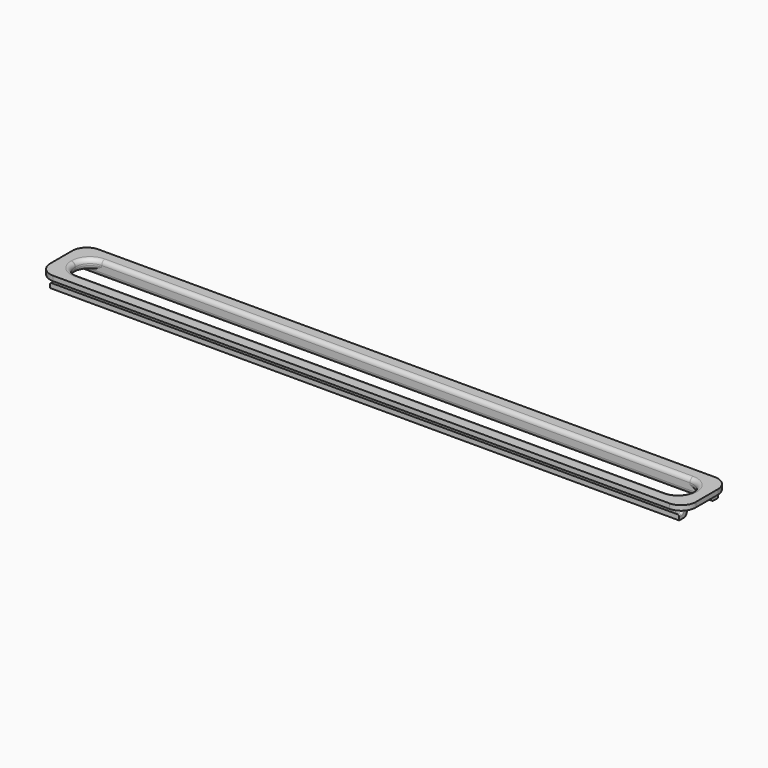
from build123d import *

# Parameters (mm, degrees)
F0_W         = 155
F0_H         = 10
F0_W_2       = 152.0637926605
F0_H_2       = 7.2836262298
F1_DEPTH     = 1.2
F2_W         = 159
F2_H         = 14
F2_W_2       = 155
F2_H_2       = 10
F2_W_3       = 152.0637926605
F2_H_3       = 7.2836262298
F3_DEPTH     = 1.2
F4_W         = 155
F4_H         = 1
F5_DEPTH     = 1.2
F6_R         = 3.6
F7_T1_DEPTH  = 160
F7_T3_DEPTH  = 0.0836262298
F7_T5_DEPTH  = 144.8637926605
F7_T10_ANGLE = 129.8047192326
F7_T13_ANGLE = 90
F7_T17_ANGLE = 129.8047192326
F7_T22_ANGLE = 129.8047192326
F7_T25_ANGLE = 90
F7_T27_ANGLE = 90
F7_T29_ANGLE = 90
F7_T33_ANGLE = 129.8047192326
F8_F1_R      = 0.5
F8_F2_R      = 0.5
F8_F3_R      = 0.5


# Not quite as in the source:
# - a fillet or chamfer that OpenCascade refuses, or shapes differently, is made with other operations: its cross-section is extruded or revolved along the edge and cut away or added


with BuildPart() as f1:
    # F0 (on Top) → F1 (new body)
    with BuildSketch(Plane.XY):
        with Locations((77.5, 5)):
            Rectangle(F0_W, F0_H)
        with Locations((77.5, 5)):
            Rectangle(F0_W_2, F0_H_2, mode=Mode.SUBTRACT)
    extrude(amount=F1_DEPTH)

    # F2 (on face) → F3 (join)
    with BuildSketch(Plane.XY.offset(1.2)):
        with Locations((77.5, 5)):
            Rectangle(F2_W, F2_H)
        with Locations((77.5, 5)):
            Rectangle(F2_W_2, F2_H_2, mode=Mode.SUBTRACT)
        with Locations((77.5, 5)):
            Rectangle(F2_W_2, F2_H_2)
        with Locations((77.5, 5)):
            Rectangle(F2_W_3, F2_H_3, mode=Mode.SUBTRACT)
    extrude(amount=F3_DEPTH)

    # F4 (on face) → F5 (join)
    with BuildSketch(Plane(origin=(0, 0, 0), x_dir=(1, 0, 0), z_dir=(0, 0, -1))):
        with Locations((77.5, 0.5)):
            Rectangle(F4_W, F4_H)
        Polygon((155, -1.3581868851), (155, 0), (0, 0), (0, -1.3581868851), (1.4681036697, -1.3581868851), (153.5318963303, -1.3581868851), align=None)
        Polygon((155, -10), (155, -8.6418131149), (153.5318963303, -8.6418131149), (1.4681036697, -8.6418131149), (0, -8.6418131149), (0, -10), align=None)
        with Locations((77.5, -10.5)):
            Rectangle(F4_W, F4_H)
    extrude(amount=F5_DEPTH)

    # F6
    f6_edges = [f1.edges().sort_by_distance(p)[0] for p in [
        (1.468104, 1.358187, 1.2),
        (1.468104, 8.641813, 1.2),
        (153.531896, 1.358187, 1.2),
        (153.531896, 8.641813, 1.2),
        (157, -2, 1.8),
        (157, 12, 1.8),
        (-2, 12, 1.8),
        (-2, -2, 1.8),
    ]]
    fillet(f6_edges, radius=F6_R)

    # F7: fillet of radius 1 on 16 edges, made by hand

    # F7_s2 → F7_t1 (cut)
    with BuildSketch(Plane.YZ.offset(-2.5)):
        with BuildLine():
            ThreePointArc((1.3581868851, -0.2), (1.0652936663, -0.9071067812), (0.3581868851, -1.2))
            Line((0.3581868851, -1.2), (1.3581868851, -1.2))
            Line((1.3581868851, -1.2), (1.3581868851, -0.2))
        make_face()
        with BuildLine():
            ThreePointArc((8.6418131149, -0.2), (8.9347063337, -0.9071067812), (9.6418131149, -1.2))
            Line((9.6418131149, -1.2), (8.6418131149, -1.2))
            Line((8.6418131149, -1.2), (8.6418131149, -0.2))
        make_face()
    extrude(amount=F7_T1_DEPTH, mode=Mode.SUBTRACT)

    # F7_s4 → F7_t3 (cut)
    with BuildSketch(Plane.XZ.offset(-5.0418131149)):
        with BuildLine():
            ThreePointArc((0.4681036697, 0), (1.1752104509, 0.2928932188), (1.4681036697, 1))
            Line((1.4681036697, 1), (1.4681036697, 0))
            Line((1.4681036697, 0), (0.4681036697, 0))
        make_face()
        with BuildLine():
            ThreePointArc((1.4681036697, 1.4), (1.1752104509, 2.1071067812), (0.4681036697, 2.4))
            Line((0.4681036697, 2.4), (1.4681036697, 2.4))
            Line((1.4681036697, 2.4), (1.4681036697, 1.4))
        make_face()
        with BuildLine():
            ThreePointArc((154.5318963303, 2.4), (153.8247895491, 2.1071067812), (153.5318963303, 1.4))
            Line((153.5318963303, 1.4), (153.5318963303, 2.4))
            Line((153.5318963303, 2.4), (154.5318963303, 2.4))
        make_face()
        with BuildLine():
            ThreePointArc((154.5318963303, 0), (153.8247895491, 0.2928932188), (153.5318963303, 1))
            Line((153.5318963303, 1), (153.5318963303, 0))
            Line((153.5318963303, 0), (154.5318963303, 0))
        make_face()
    extrude(amount=F7_T3_DEPTH, mode=Mode.SUBTRACT)

    # F7_s6 → F7_t5 (cut)
    with BuildSketch(Plane.YZ.offset(5.0681036697)):
        with BuildLine():
            ThreePointArc((1.3581868851, 1.4), (1.0652936663, 2.1071067812), (0.3581868851, 2.4))
            Line((0.3581868851, 2.4), (1.3581868851, 2.4))
            Line((1.3581868851, 2.4), (1.3581868851, 1.4))
        make_face()
        with BuildLine():
            ThreePointArc((8.6418131149, 1.4), (8.9347063337, 2.1071067812), (9.6418131149, 2.4))
            Line((9.6418131149, 2.4), (8.6418131149, 2.4))
            Line((8.6418131149, 2.4), (8.6418131149, 1.4))
        make_face()
    extrude(amount=F7_T5_DEPTH, mode=Mode.SUBTRACT)


with BuildPart() as f7_tool8:
    # F7_s9 → F7_t10 (revolve)
    with BuildSketch(Plane(origin=(0.5115194158, -0.4262532935, 0), x_dir=(0, 0, 1), z_dir=(0.7682307976, -0.6401729779, 0))):
        with BuildLine():
            ThreePointArc((0, -11.7177391291), (0.2928932188, -11.0106323479), (1, -10.7177391291))
            Line((1, -10.7177391291), (0, -10.7177391291))
            Line((0, -10.7177391291), (0, -11.7177391291))
        make_face()
    revolve(axis=Axis((5.0681036697, 5.0418131149, 0), (0, 0, 1)), revolution_arc=F7_T10_ANGLE)

    split(bisect_by=Plane.XZ.offset(-8.6418131149), keep=Keep.TOP)


with BuildPart() as f1_1:
    add(f1.part)

    # F7_t7: cut F7_tool8
    add(f7_tool8.part, mode=Mode.SUBTRACT)

    # F7_s12 → F7_t13 (revolve, cut)
    with BuildSketch(Plane.YZ.offset(5.0681036697)):
        with BuildLine():
            ThreePointArc((8.6418131149, 1.4), (8.9347063337, 2.1071067812), (9.6418131149, 2.4))
            Line((9.6418131149, 2.4), (8.6418131149, 2.4))
            Line((8.6418131149, 2.4), (8.6418131149, 1.4))
        make_face()
    revolve(axis=Axis((5.0681036697, 5.0418131149, 2.4), (0, 0, 1)), revolution_arc=F7_T13_ANGLE, mode=Mode.SUBTRACT)


with BuildPart() as f7_tool15:
    # F7_s16 → F7_t17 (revolve)
    with BuildSketch(Plane(origin=(90.9661571375, 75.8028393036, 0), x_dir=(0, 0, 1), z_dir=(-0.7682307976, -0.6401729779, 0))):
        with BuildLine():
            ThreePointArc((0, -87.5090724404), (0.2928932188, -88.2161792216), (1, -88.5090724404))
            Line((1, -88.5090724404), (0, -88.5090724404))
            Line((0, -88.5090724404), (0, -87.5090724404))
        make_face()
    revolve(axis=Axis((149.9318963303, 5.0418131149, 0), (0, 0, -1)), revolution_arc=F7_T17_ANGLE)

    split(bisect_by=Plane.XZ.offset(-8.6418131149), keep=Keep.TOP)


with BuildPart() as f1_2:
    add(f1_1.part)

    # F7_t14: cut F7_tool15
    add(f7_tool15.part, mode=Mode.SUBTRACT)


with BuildPart() as f7_tool20:
    # F7_s21 → F7_t22 (revolve)
    with BuildSketch(Plane.XZ.offset(-4.9581868851)):
        with BuildLine():
            ThreePointArc((0.4681036697, 0), (1.1752104509, 0.2928932188), (1.4681036697, 1))
            Line((1.4681036697, 1), (1.4681036697, 0))
            Line((1.4681036697, 0), (0.4681036697, 0))
        make_face()
    revolve(axis=Axis((5.0681036697, 4.9581868851, 0), (0, 0, 1)), revolution_arc=F7_T22_ANGLE)

    split(bisect_by=Plane.XZ.offset(-1.3581868851), keep=Keep.BOTTOM)


with BuildPart() as f1_3:
    add(f1_2.part)

    # F7_t19: cut F7_tool20
    add(f7_tool20.part, mode=Mode.SUBTRACT)

    # F7_s24 → F7_t25 (revolve, cut)
    with BuildSketch(Plane.XZ.offset(-4.9581868851)):
        with BuildLine():
            ThreePointArc((1.4681036697, 1.4), (1.1752104509, 2.1071067812), (0.4681036697, 2.4))
            Line((0.4681036697, 2.4), (1.4681036697, 2.4))
            Line((1.4681036697, 2.4), (1.4681036697, 1.4))
        make_face()
    revolve(axis=Axis((5.0681036697, 4.9581868851, 2.4), (0, 0, 1)), revolution_arc=F7_T25_ANGLE, mode=Mode.SUBTRACT)

    # F7_s26 → F7_t27 (revolve, cut)
    with BuildSketch(Plane.YZ.offset(149.9318963303)):
        with BuildLine():
            ThreePointArc((9.6418131149, 2.4), (8.9347063337, 2.1071067812), (8.6418131149, 1.4))
            Line((8.6418131149, 1.4), (8.6418131149, 2.4))
            Line((8.6418131149, 2.4), (9.6418131149, 2.4))
        make_face()
    revolve(axis=Axis((149.9318963303, 5.0418131149, 2.4), (0, 0, -1)), revolution_arc=F7_T27_ANGLE, mode=Mode.SUBTRACT)

    # F7_s28 → F7_t29 (revolve, cut)
    with BuildSketch(Plane.YZ.offset(149.9318963303)):
        with BuildLine():
            ThreePointArc((0.3581868851, 2.4), (1.0652936663, 2.1071067812), (1.3581868851, 1.4))
            Line((1.3581868851, 1.4), (1.3581868851, 2.4))
            Line((1.3581868851, 2.4), (0.3581868851, 2.4))
        make_face()
    revolve(axis=Axis((149.9318963303, 4.9581868851, 2.4), (0, 0, 1)), revolution_arc=F7_T29_ANGLE, mode=Mode.SUBTRACT)


with BuildPart() as f7_tool31:
    # F7_s32 → F7_t33 (revolve)
    with BuildSketch(Plane(origin=(86.0481511635, -71.7046248877, 0), x_dir=(0, 0, 1), z_dir=(-0.7682307976, 0.6401729779, 0))):
        with BuildLine():
            ThreePointArc((1, 96.1913804165), (0.2928932188, 95.8984871977), (0, 95.1913804165))
            Line((0, 95.1913804165), (0, 96.1913804165))
            Line((0, 96.1913804165), (1, 96.1913804165))
        make_face()
    revolve(axis=Axis((149.9318963303, 4.9581868851, 0), (0, 0, 1)), revolution_arc=F7_T33_ANGLE)

    split(bisect_by=Plane.XZ.offset(-1.3581868851), keep=Keep.BOTTOM)


with BuildPart() as f1_4:
    add(f1_3.part)

    # F7_t30: cut F7_tool31
    add(f7_tool31.part, mode=Mode.SUBTRACT)

    # F8: fillet of radius 0.5 on 10 edges, made by hand

    # F8_f1
    f8_f1_edges = [f1_4.edges().sort_by_distance(p)[0] for p in [
        (77.5, 0, 0),
        (77.5, 10, 0),
    ]]
    fillet(f8_f1_edges, radius=F8_F1_R)

    # F8_f2
    f8_f2_edges = [f1_4.edges().sort_by_distance(p)[0] for p in [
        (0, 0, 0.85),
        (155, 0, 0.85),
        (155, 10, 0.85),
        (0, 10, 0.85),
        (0, 10.1464466094, 0.1464466094),
        (155, 10.1464466094, 0.1464466094),
        (155, -0.1464466094, 0.1464466094),
        (0, -0.1464466094, 0.1464466094),
    ]]
    fillet(f8_f2_edges, radius=F8_F2_R)

    # F8_f3
    f8_f3_edges = [f1_4.edges().sort_by_distance(p)[0] for p in [
        (77.5, 0, 1.2),
        (77.5, 10, 1.2),
        (155, 5, 1.2),
        (0, 5, 1.2),
        (0.1464466094, 9.8535533906, 1.2),
        (0.1464466094, 0.1464466094, 1.2),
        (154.8535533906, 0.1464466094, 1.2),
        (154.8535533906, 9.8535533906, 1.2),
    ]]
    fillet(f8_f3_edges, radius=F8_F3_R)


solid = f1_4.part
